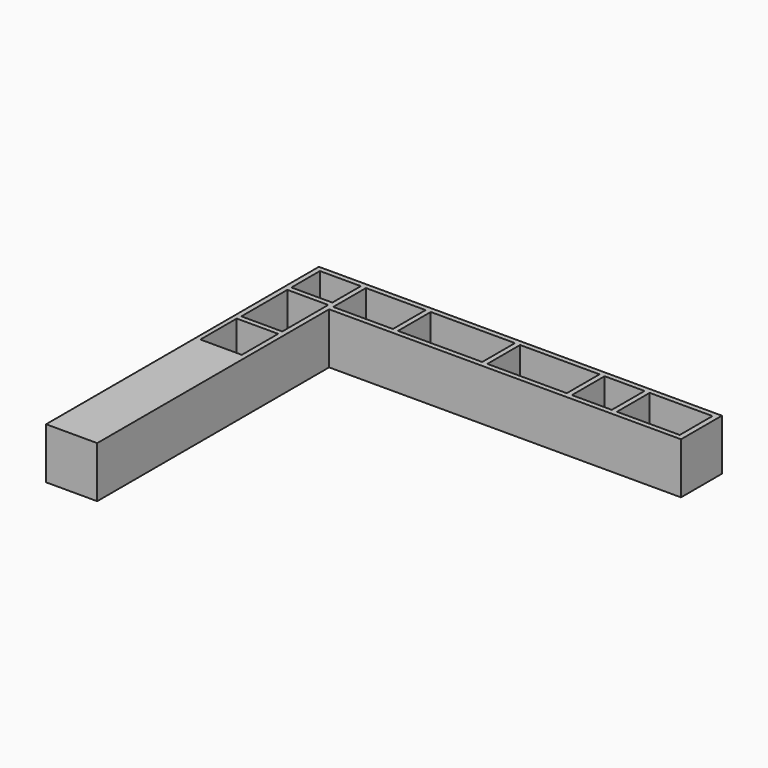
from build123d import *

# Parameters (mm, degrees)
F0_W     = 2064
F0_H     = 300
F1_DEPTH = 300
F2_W     = 243.0647516251
F2_H     = 266.6307017207
F2_W_2   = 240
F2_H_2   = 337.1192961931
F2_H_3   = 208.7436437607
F2_W_3   = 350.139864234
F2_H_4   = 240
F2_W_4   = 494.0672528744
F2_W_5   = 465.8082723618
F2_W_6   = 234.2424714565
F2_W_7   = 368.4137177467
F3_DEPTH = 280


# Not quite as in the source:
# - a feature names something its author has since deleted; it is built from what else it names


with BuildPart() as f1:
    # F0 (on Top) → F1 (new body)
    with BuildSketch(Plane.XY):
        Polygon((-1332.5527270117, 866.6404155501), (-1332.5527270117, -1133.3595844499), (-1032.5527270117, -1133.3595844499), (-1032.5527270117, 566.6404155501), (-1032.5527270117, 866.6404155501), align=None)
        with Locations((-0.5527270117, 716.6404155501)):
            Rectangle(F0_W, F0_H)
    extrude(amount=F1_DEPTH)

    # F2 (on face) → F3 (cut)
    with BuildSketch(Plane.XY.offset(300)):
        with Locations((-1184.0851028242, 97.462124736)):
            Rectangle(F2_W, F2_H)
        with Locations((-1182.5527270117, 429.3371236929)):
            Rectangle(F2_W_2, F2_H_2)
        with Locations((-1182.5527270117, 732.2685936698)):
            Rectangle(F2_W_2, F2_H_3)
        with Locations((-857.4827948947, 716.6404155501)):
            Rectangle(F2_W_3, F2_H_4)
        with Locations((-405.3792363405, 716.6404155501)):
            Rectangle(F2_W_4, F2_H_4)
        with Locations((104.5585262775, 716.6404155501)):
            Rectangle(F2_W_5, F2_H_4)
        with Locations((484.5838981867, 716.6404155501)):
            Rectangle(F2_W_6, F2_H_4)
        with Locations((815.9119927883, 716.6404155501)):
            Rectangle(F2_W_7, F2_H_4)
    extrude(amount=-F3_DEPTH, mode=Mode.SUBTRACT)


solid = f1.part
